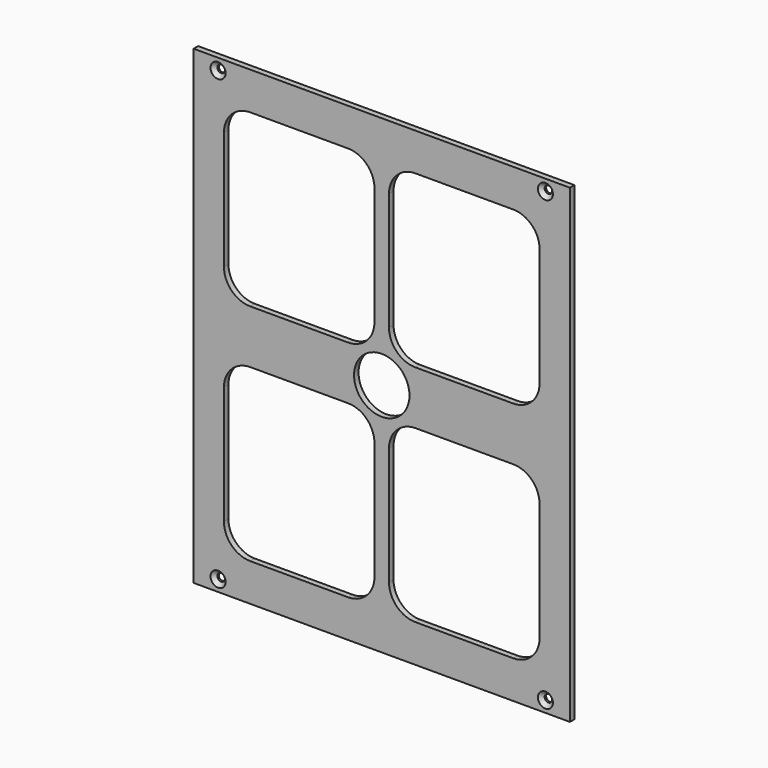
from build123d import *

# Parameters (mm, degrees)
F0_W           = 100
F0_H           = 125
F0_R           = 7.3677826157
F1_DEPTH       = 1.5
F3_D           = 2
F3_CSINK_D     = 4
F3_CSINK_ANGLE = 90


# Not quite as in the source:
# - a feature names something its author has since deleted; it is built from what else it names


with BuildPart() as f1:
    # F0 (on Front) → F1 (new body)
    with BuildSketch(Plane.XZ):
        Rectangle(F0_W, F0_H)
        with BuildLine():
            Line((-34.9434472264, -7.1068441343), (-8.9434472264, -7.1068441343))
            ThreePointArc((-8.9434472264, -7.1068441343), (-3.9936997581, -9.157096666), (-1.9434472264, -14.1068441343))
            Line((-1.9434472264, -14.1068441343), (-1.9434472264, -45.5))
            ThreePointArc((-1.9434472264, -45.5), (-3.9936997581, -50.4497474683), (-8.9434472264, -52.5))
            Line((-8.9434472264, -52.5), (-34.9434472264, -52.5))
            ThreePointArc((-34.9434472264, -52.5), (-39.8931946947, -50.4497474683), (-41.9434472264, -45.5))
            Line((-41.9434472264, -45.5), (-41.9434472264, -14.1068441343))
            ThreePointArc((-41.9434472264, -14.1068441343), (-39.8931946947, -9.157096666), (-34.9434472264, -7.1068441343))
        make_face(mode=Mode.SUBTRACT)
        with BuildLine():
            ThreePointArc((41.9434472264, -45.5), (39.8931946947, -50.4497474683), (34.9434472264, -52.5))
            Line((34.9434472264, -52.5), (8.9434472264, -52.5))
            ThreePointArc((8.9434472264, -52.5), (3.9936997581, -50.4497474683), (1.9434472264, -45.5))
            Line((1.9434472264, -45.5), (1.9434472264, -14.1068441343))
            ThreePointArc((1.9434472264, -14.1068441343), (3.9936997581, -9.157096666), (8.9434472264, -7.1068441343))
            Line((8.9434472264, -7.1068441343), (34.9434472264, -7.1068441343))
            ThreePointArc((34.9434472264, -7.1068441343), (39.8931946947, -9.157096666), (41.9434472264, -14.1068441343))
            Line((41.9434472264, -14.1068441343), (41.9434472264, -45.5))
        make_face(mode=Mode.SUBTRACT)
        with BuildLine():
            ThreePointArc((-1.9434472264, 14.1068441343), (-3.9936997581, 9.157096666), (-8.9434472264, 7.1068441343))
            Line((-8.9434472264, 7.1068441343), (-34.9434472264, 7.1068441343))
            ThreePointArc((-34.9434472264, 7.1068441343), (-39.8931946947, 9.157096666), (-41.9434472264, 14.1068441343))
            Line((-41.9434472264, 14.1068441343), (-41.9434472264, 45.5))
            ThreePointArc((-41.9434472264, 45.5), (-39.8931946947, 50.4497474683), (-34.9434472264, 52.5))
            Line((-34.9434472264, 52.5), (-8.9434472264, 52.5))
            ThreePointArc((-8.9434472264, 52.5), (-3.9936997581, 50.4497474683), (-1.9434472264, 45.5))
            Line((-1.9434472264, 45.5), (-1.9434472264, 14.1068441343))
        make_face(mode=Mode.SUBTRACT)
        Circle(F0_R, mode=Mode.SUBTRACT)
        with BuildLine():
            ThreePointArc((8.9434472264, 7.1068441343), (3.9936997581, 9.157096666), (1.9434472264, 14.1068441343))
            Line((1.9434472264, 14.1068441343), (1.9434472264, 45.5))
            ThreePointArc((1.9434472264, 45.5), (3.9936997581, 50.4497474683), (8.9434472264, 52.5))
            Line((8.9434472264, 52.5), (34.9434472264, 52.5))
            ThreePointArc((34.9434472264, 52.5), (39.8931946947, 50.4497474683), (41.9434472264, 45.5))
            Line((41.9434472264, 45.5), (41.9434472264, 14.1068441343))
            ThreePointArc((41.9434472264, 14.1068441343), (39.8931946947, 9.157096666), (34.9434472264, 7.1068441343))
            Line((34.9434472264, 7.1068441343), (8.9434472264, 7.1068441343))
        make_face(mode=Mode.SUBTRACT)
    extrude(amount=F1_DEPTH)

    # F3 (through all)
    with Locations(Plane.XZ.offset(1.5)):
        with Locations((-43.5, -59.5), (43.5, -59.5), (43.5, 59.5), (-43.5, 59.5)):
            CounterSinkHole(F3_D / 2, F3_CSINK_D / 2, counter_sink_angle=F3_CSINK_ANGLE)


solid = f1.part
